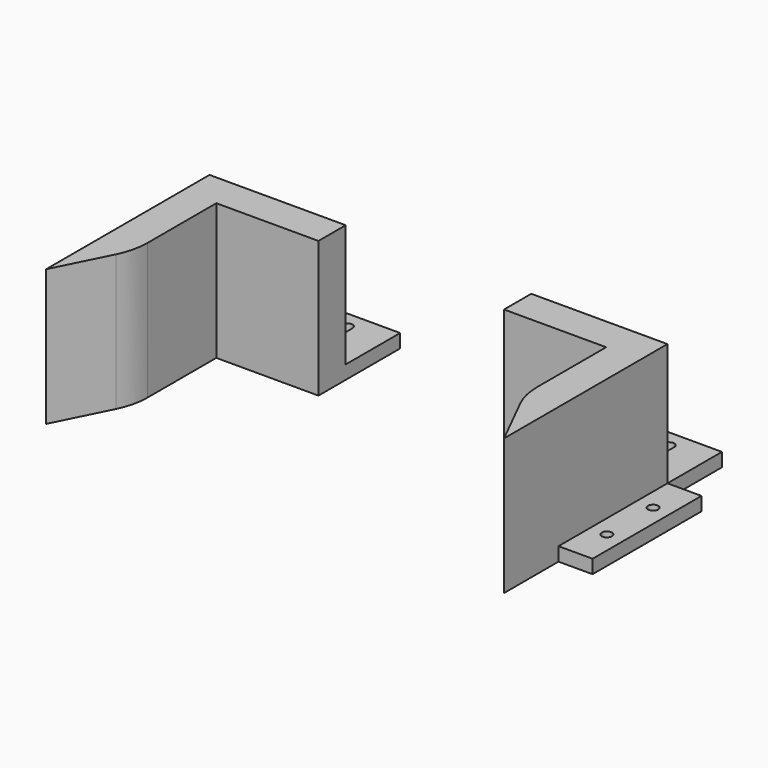
from build123d import *

# Parameters (mm, degrees)
F1_DEPTH = 4
F0_W     = 10
F0_H     = 40
F0_R     = 1.5
F0_W_2   = 30
F0_H_2   = 10
F2_DEPTH = 40
F3_R     = 20
F3_2_R   = 20


# Not quite as in the source:
# - a feature names something its author has since deleted; it is built from what else it names


with BuildPart() as f1:
    # F0 (on Top) → F1 (new body)
    with BuildSketch(Plane.XY):
        Polygon((-30, 30), (-30, 10), (0, 10), (10, 10), (10, 30), align=None)
        with BuildLine():
            Line((-20, 15), (-20, 25))
            ThreePointArc((-20, 25), (-18.5, 26.5), (-17, 25))
            Line((-17, 25), (-17, 15))
            ThreePointArc((-17, 15), (-18.5, 13.5), (-20, 15))
        make_face(mode=Mode.SUBTRACT)
        with BuildLine():
            Line((-3, 15), (-3, 25))
            ThreePointArc((-3, 25), (-1.5, 26.5), (0, 25))
            Line((0, 25), (0, 15))
            ThreePointArc((0, 15), (-1.5, 13.5), (-3, 15))
        make_face(mode=Mode.SUBTRACT)
    extrude(amount=F1_DEPTH)



with BuildPart() as f1b:
    # F0 (on Top) → F1, piece 2 (new body)
    with BuildSketch(Plane.XY):
        with Locations((15, -10)):
            Rectangle(F0_W, F0_H)
        with Locations((15, -18.5)):
            Circle(F0_R, mode=Mode.SUBTRACT)
        with Locations((15, -1.5)):
            Circle(F0_R, mode=Mode.SUBTRACT)
    extrude(amount=F1_DEPTH)


with BuildPart() as f1c:
    # F0 (on Top) → F1, piece 3 (new body)
    with BuildSketch(Plane.XY):
        Polygon((-84.5099326968, 30), (-124.5099326968, 30), (-124.5099326968, 10), (-114.5099326968, 10), (-84.5099326968, 10), align=None)
        with BuildLine():
            Line((-111.5099326968, 25), (-111.5099326968, 15))
            ThreePointArc((-111.5099326968, 15), (-113.0099326968, 13.5), (-114.5099326968, 15))
            Line((-114.5099326968, 15), (-114.5099326968, 25))
            ThreePointArc((-114.5099326968, 25), (-113.0099326968, 26.5), (-111.5099326968, 25))
        make_face(mode=Mode.SUBTRACT)
        with BuildLine():
            Line((-97.5099326968, 15), (-97.5099326968, 25))
            ThreePointArc((-97.5099326968, 25), (-96.0099326968, 26.5), (-94.5099326968, 25))
            Line((-94.5099326968, 25), (-94.5099326968, 15))
            ThreePointArc((-94.5099326968, 15), (-96.0099326968, 13.5), (-97.5099326968, 15))
        make_face(mode=Mode.SUBTRACT)
    extrude(amount=F1_DEPTH)



with BuildPart() as f1d:
    # F0 (on Top) → F1, piece 4 (new body)
    with BuildSketch(Plane.XY):
        with Locations((-129.5099326968, -10)):
            Rectangle(F0_W, F0_H)
        with Locations((-129.5099326968, -18.5)):
            Circle(F0_R, mode=Mode.SUBTRACT)
        with Locations((-129.5099326968, -1.5)):
            Circle(F0_R, mode=Mode.SUBTRACT)
    extrude(amount=F1_DEPTH)


with BuildPart() as f1_1:
    add(f1.part)

    add(f1b.part)  # F2 merges F1b
    # F0 (on Top) → F2 (join)
    with BuildSketch(Plane.XY):
        with Locations((-15, 5)):
            Rectangle(F0_W_2, F0_H_2)
        Polygon((10, 10), (0, 10), (0, 0), (0, -30), (10, -30), align=None)
        Polygon((10, -30), (0, -30), (10, -50), align=None)
    extrude(amount=F2_DEPTH)

    # F3
    f3_edges = [f1_1.edges().sort_by_distance(p)[0] for p in [
        (0, -30, 20),
    ]]
    fillet(f3_edges, radius=F3_R)


with BuildPart() as f1c_1:
    add(f1c.part)

    add(f1d.part)  # F2#2 merges F1d
    # F0 (on Top) → F2, piece 2 (join)
    with BuildSketch(Plane.XY):
        with Locations((-99.5099326968, 5)):
            Rectangle(F0_W_2, F0_H_2)
        Polygon((-114.5099326968, 10), (-124.5099326968, 10), (-124.5099326968, -30), (-114.5099326968, -30), (-114.5099326968, 0), align=None)
        Polygon((-114.5099326968, -30), (-124.5099326968, -30), (-124.5099326968, -50), align=None)
    extrude(amount=F2_DEPTH)

    # F3#2
    f3_2_edges = [f1c_1.edges().sort_by_distance(p)[0] for p in [
        (-114.509933, -30, 20),
    ]]
    fillet(f3_2_edges, radius=F3_2_R)


solid = Compound([f1_1.part, f1c_1.part])
